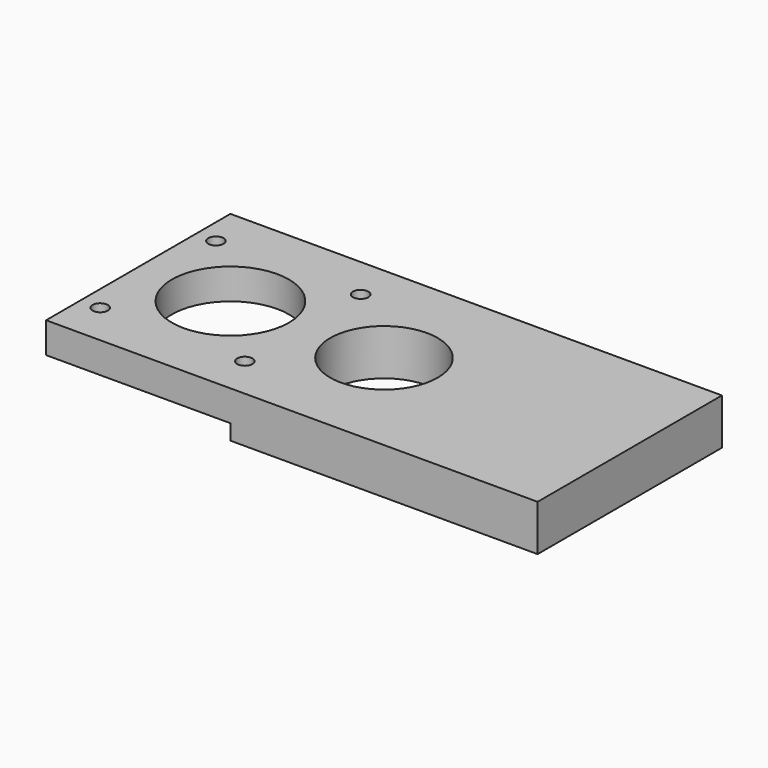
from build123d import *

# Parameters (mm, degrees)
F0_W     = 160
F0_H     = 75
F0_R     = 17.5
F1_DEPTH = 15
F2_R     = 2.5
F2_R_2   = 19.05
F3_DEPTH = 25
F4_R     = 4
F5_DEPTH = 6
F6_W     = 60
F6_H     = 5
F7_DEPTH = 79.7


# Not quite as in the source:
# - a feature names something its author has since deleted; it is built from what else it names


with BuildPart() as f1:
    # F0 (on Top) → F1 (new body)
    with BuildSketch(Plane.XY):
        Rectangle(F0_W, F0_H)
        Circle(F0_R, mode=Mode.SUBTRACT)
    extrude(amount=F1_DEPTH)

    # F2 (on face) → F3 (cut)
    with BuildSketch(Plane.XY.offset(15)):
        with Locations((-73.55, 23.55)):
            Circle(F2_R)
        with Locations((-26.45, 23.55)):
            Circle(F2_R)
        with Locations((-26.45, -23.55)):
            Circle(F2_R)
        with Locations((-73.55, -23.55)):
            Circle(F2_R)
        with Locations((-50, 0)):
            Circle(F2_R_2)
    extrude(amount=-F3_DEPTH, mode=Mode.SUBTRACT)

    # F4 (on face) → F5 (cut)
    with BuildSketch(Plane(origin=(0, 0, 0), x_dir=(1, 0, 0), z_dir=(0, 0, -1))):
        with Locations((-73.55, 23.55)):
            Circle(F4_R)
        with Locations((-26.45, 23.55)):
            Circle(F4_R)
        with Locations((-26.45, -23.55)):
            Circle(F4_R)
        with Locations((-73.55, -23.55)):
            Circle(F4_R)
    extrude(amount=-F5_DEPTH, mode=Mode.SUBTRACT)

    # F6 (on face) → F7 (cut)
    with BuildSketch(Plane.XZ.offset(37.5)):
        with Locations((-50, 2.5)):
            Rectangle(F6_W, F6_H)
    extrude(amount=-F7_DEPTH, mode=Mode.SUBTRACT)


solid = f1.part
